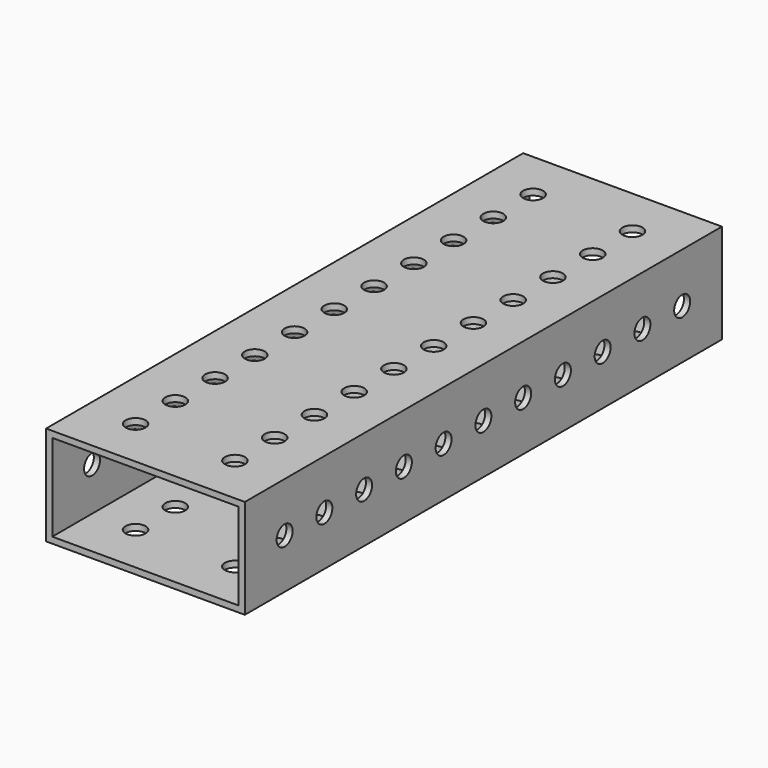
from build123d import *

# Parameters (mm, degrees)
F0_W     = 50.8
F0_H     = 25.4
F0_W_2   = 47.625
F0_H_2   = 22.225
F1_DEPTH = 152.4
F2_R     = 2.5527
F3_DEPTH = 50.8
F4_R     = 2.5527
F5_DEPTH = 254


# Not quite as in the source:
# - a feature names something its author has since deleted; it is built from what else it names


with BuildPart() as f1:
    # F0 (on Front) → F1 (new body)
    with BuildSketch(Plane.XZ):
        Rectangle(F0_W, F0_H)
        Rectangle(F0_W_2, F0_H_2, mode=Mode.SUBTRACT)
    extrude(amount=F1_DEPTH)

    # F2 (on face) → F3 (cut)
    with BuildSketch(Plane(origin=(-25.4, 0, 0), x_dir=(0, -1, 0), z_dir=(-1, 0, 0))):
        with Locations((139.7, 0)):
            Circle(F2_R)
        with Locations((114.3, 0)):
            Circle(F2_R)
        with Locations((25.4, 0)):
            Circle(F2_R)
        with Locations((101.6, 0)):
            Circle(F2_R)
        with Locations((88.9, 0)):
            Circle(F2_R)
        with Locations((127, 0)):
            Circle(F2_R)
        with Locations((63.5, 0)):
            Circle(F2_R)
        with Locations((76.2, 0)):
            Circle(F2_R)
        with Locations((12.7, 0)):
            Circle(F2_R)
        with Locations((38.1, 0)):
            Circle(F2_R)
        with Locations((50.8, 0)):
            Circle(F2_R)
    extrude(amount=-F3_DEPTH, mode=Mode.SUBTRACT)

    # F4 (on face) → F5 (cut)
    with BuildSketch(Plane(origin=(0, 0, -12.7), x_dir=(1, 0, 0), z_dir=(0, 0, -1))):
        with Locations((12.7, 114.3)):
            Circle(F4_R)
        with Locations((-12.7, 12.7)):
            Circle(F4_R)
        with Locations((12.7, 76.2)):
            Circle(F4_R)
        with Locations((-12.7, 25.4)):
            Circle(F4_R)
        with Locations((12.7, 139.7)):
            Circle(F4_R)
        with Locations((12.7, 50.8)):
            Circle(F4_R)
        with Locations((-12.7, 101.6)):
            Circle(F4_R)
        with Locations((-12.7, 50.8)):
            Circle(F4_R)
        with Locations((12.7, 101.6)):
            Circle(F4_R)
        with Locations((12.7, 12.7)):
            Circle(F4_R)
        with Locations((12.7, 88.9)):
            Circle(F4_R)
        with Locations((-12.7, 127)):
            Circle(F4_R)
        with Locations((12.7, 127)):
            Circle(F4_R)
        with Locations((-12.7, 76.2)):
            Circle(F4_R)
        with Locations((-12.7, 139.7)):
            Circle(F4_R)
        with Locations((-12.7, 88.9)):
            Circle(F4_R)
        with Locations((-12.7, 38.1)):
            Circle(F4_R)
        with Locations((12.7, 38.1)):
            Circle(F4_R)
        with Locations((12.7, 63.5)):
            Circle(F4_R)
        with Locations((-12.7, 114.3)):
            Circle(F4_R)
        with Locations((-12.7, 63.5)):
            Circle(F4_R)
        with Locations((12.7, 25.4)):
            Circle(F4_R)
    extrude(amount=-F5_DEPTH, mode=Mode.SUBTRACT)


solid = f1.part
